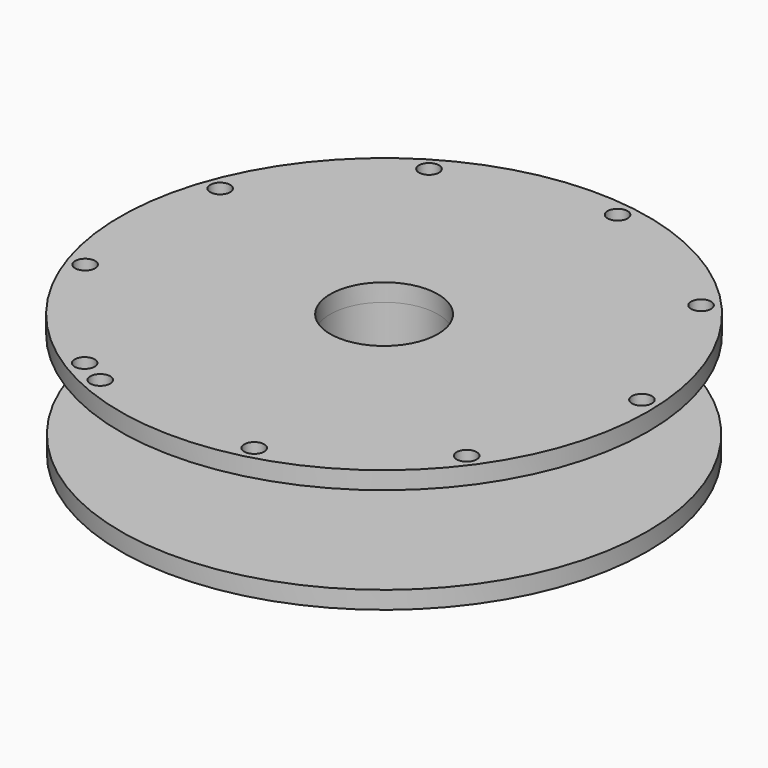
from build123d import *

# Parameters (mm, degrees)
F0_R     = 29.9089661925
F1_DEPTH = 2
F2_R     = 10.0009924636
F3_DEPTH = 10
F4_R     = 29.9764800093
F5_DEPTH = 2
F6_R     = 1.1365848363
F7_DEPTH = 25
F8_R     = 6.1187155748
F9_DEPTH = 25


with BuildPart() as f1:
    # F0 (on Top) → F1 (new body)
    with BuildSketch(Plane.XY):
        Circle(F0_R)
    extrude(amount=F1_DEPTH)

    # F2 (on face) → F3 (join)
    with BuildSketch(Plane.XY.offset(2)):
        Circle(F2_R)
    extrude(amount=F3_DEPTH)


with BuildPart() as f5:
    # F4 (on face) → F5 (new body)
    with BuildSketch(Plane.XY.offset(12)):
        Circle(F4_R)
    extrude(amount=F5_DEPTH)

    # F6 (on face) → F7 (cut)
    with BuildSketch(Plane.XY.offset(14)):
        with Locations((-14.8717621341, -23.9195972681)):
            Circle(F6_R)
        with Locations((-26.6426764835, -9.136970627)):
            Circle(F6_R)
        with Locations((-26.4214284802, 9.7583072051)):
            Circle(F6_R)
        with Locations((-14.3076042892, 24.2612634038)):
            Circle(F6_R)
        with Locations((4.2462302972, 27.8439575259)):
            Circle(F6_R)
        with Locations((20.888789823, 18.8937794571)):
            Circle(F6_R)
        with Locations((28.1290748038, 1.439302999)):
            Circle(F6_R)
        with Locations((22.7081531643, -16.6630196036)):
            Circle(F6_R)
        with Locations((7.0660414861, -27.2651334154)):
            Circle(F6_R)
        with Locations((-11.75657335, -25.5949101485)):
            Circle(F6_R)
    extrude(amount=-F7_DEPTH, mode=Mode.SUBTRACT)


with BuildPart() as f9_tool:
    # F8 (on face) → F9 (new body)
    with BuildSketch(Plane.XY.offset(14)):
        Circle(F8_R)
    extrude(amount=-F9_DEPTH)


with BuildPart() as f1_1:
    add(f1.part)

    # F9: cut by f9_tool
    add(f9_tool.part, mode=Mode.SUBTRACT)


with BuildPart() as f5_1:
    add(f5.part)

    # F9: cut by f9_tool
    add(f9_tool.part, mode=Mode.SUBTRACT)


solid = Compound([f1_1.part, f5_1.part])
